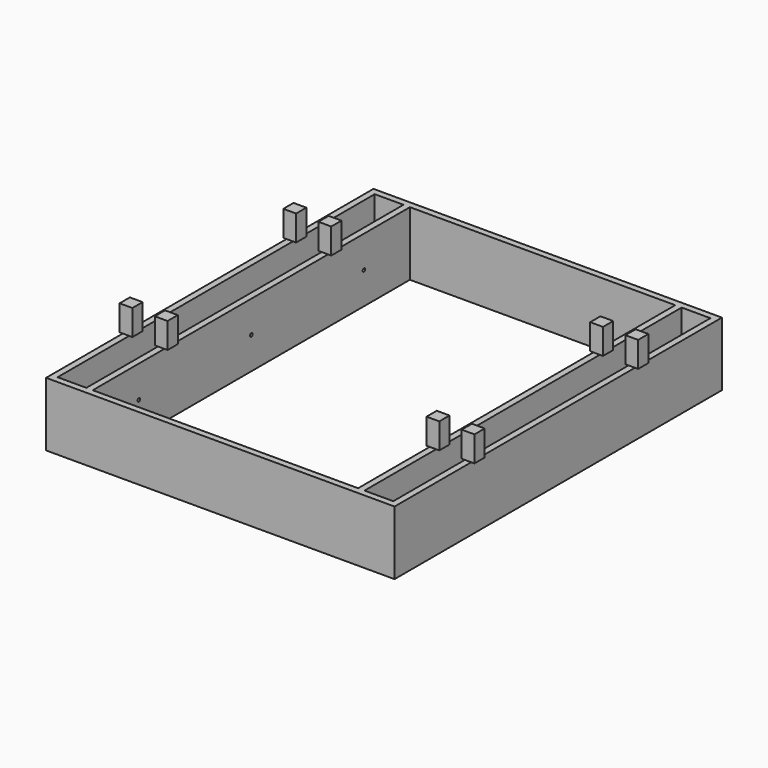
from build123d import *

# Parameters (mm, degrees)
F1_DEPTH = 63.5
F2_R     = 3.175
F3_DEPTH = 12.7
F6_DEPTH = 12.7


# Not quite as in the source:
# - a pattern or mirror of a feature is missing from the dataset's text; its kind, count and spacing are read off the source's solid


with BuildPart() as f1:
    # F0 (on Top) → F1 (new body, symmetric)
    with BuildSketch(Plane.XY):
        Polygon((-346.075, -406.4), (346.075, -406.4), (346.075, -393.7), (346.075, 406.4), (-290.28644, 406.4), (-294.2266940207, 406.4), (-346.075, 406.4), (-346.075, 393.7), align=None)
        Polygon((-276.225, 393.7), (-276.225, 383.1179738045), (-276.225, -393.7), (-333.375, -393.7), (-333.375, 393.7), align=None, mode=Mode.SUBTRACT)
        Polygon((-263.525, -393.7), (-263.525, 383.1179738045), (-263.525, 393.7), (263.525, 393.7), (263.525, 383.1179738045), (263.525, -393.7), align=None, mode=Mode.SUBTRACT)
        Polygon((333.375, 393.7), (333.375, -393.7), (276.225, -393.7), (276.225, 383.1179738045), (276.225, 393.7), align=None, mode=Mode.SUBTRACT)
    extrude(amount=F1_DEPTH, both=True)

    # F2 (on face) → F3 (cut)
    with BuildSketch(Plane(origin=(263.525, 0, 0), x_dir=(0, -1, 0), z_dir=(-1, 0, 0))):
        Circle(F2_R)
        with Locations((-279.4, 0)):
            Circle(F2_R)
        with Locations((279.4, 0)):
            Circle(F2_R)
    f3 = extrude(amount=-F3_DEPTH, mode=Mode.SUBTRACT)

    # F3_copies: F3 across plane
    add(f3.mirror(Plane(origin=(0, 0, 0), x_dir=(0, 0, -1), z_dir=(-1, 0, 0))), mode=Mode.SUBTRACT)

    # F5 (on mid) → F6 (join, symmetric)
    with BuildSketch(Plane.YZ.offset(339.725)):
        Polygon((-215.9, 63.5), (-203.2, 63.5), (-190.5, 63.5), (-190.5, 114.3), (-215.9, 114.3), align=None)
        Polygon((190.5, 63.5), (203.2, 63.5), (215.9, 63.5), (215.9, 114.3), (190.5, 114.3), align=None)
    f6 = extrude(amount=F6_DEPTH, both=True)

    # F6_copies: F6 across plane
    add(f6.mirror(Plane(origin=(0, 0, 0), x_dir=(0, 0, -1), z_dir=(-1, 0, 0))))

    # F6_copies1: F6 across plane
    add(f6.mirror(Plane(origin=(304.8, 0, 0), x_dir=(0, 0, -1), z_dir=(-1, 0, 0))))

    # F6_copies2: F6 across plane
    add(f6.mirror(Plane(origin=(34.925, 0, 0), x_dir=(0, 0, -1), z_dir=(-1, 0, 0))))


solid = f1.part
